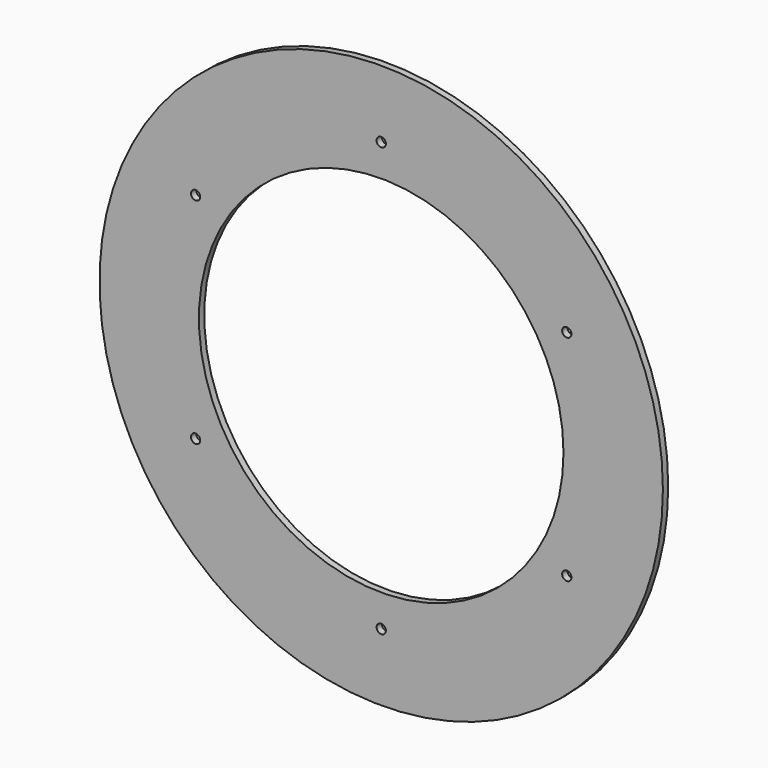
from build123d import *

# Parameters (mm, degrees)
F0_R            = 127.5
F0_R_2          = 82.5
F1_DEPTH        = 3
F2_R            = 2.1
F3_DEPTH        = 3
F3_COPIES_COUNT = 6


# Not quite as in the source:
# - a pattern or mirror of a feature is missing from the dataset's text; its kind, count and spacing are read off the source's solid


with BuildPart() as f1:
    # F0 (on Front) → F1 (new body)
    with BuildSketch(Plane.XZ):
        Circle(F0_R)
        Circle(F0_R_2, mode=Mode.SUBTRACT)
    extrude(amount=F1_DEPTH)

    # F2 (on face) → F3 (cut, through all)
    with BuildSketch(Plane.XZ.offset(3)):
        with Locations((0, 97)):
            Circle(F2_R)
    f3 = extrude(amount=-F3_DEPTH, mode=Mode.SUBTRACT)

    # F3_copies: F3 ×6 about axis
    f3_copies_axis = Axis((0, 0, 0), (0, 1, 0))
    for i in range(1, F3_COPIES_COUNT):
        add(f3.rotate(f3_copies_axis, i * 360 / F3_COPIES_COUNT), mode=Mode.SUBTRACT)


solid = f1.part
